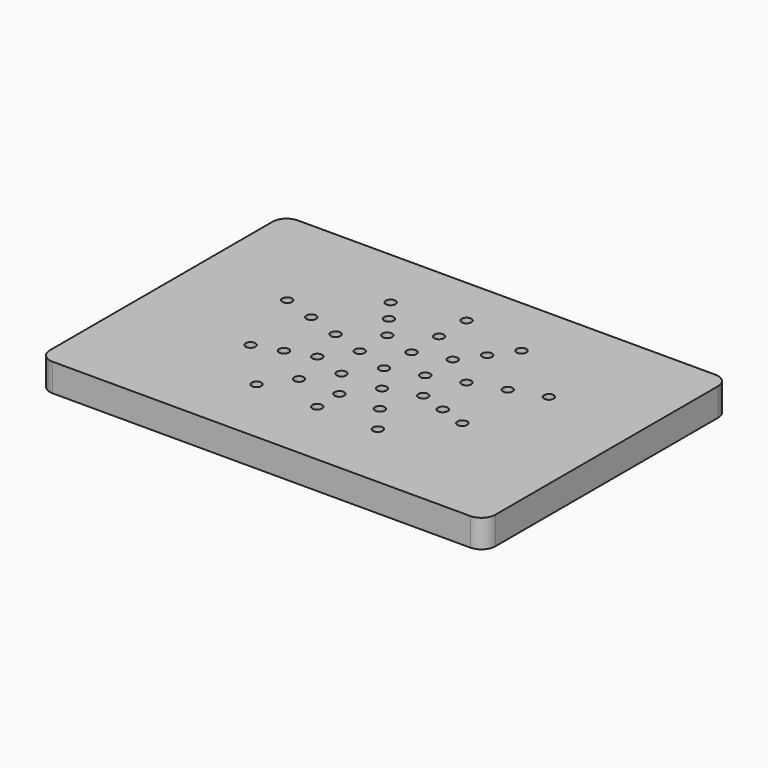
from build123d import *

# Parameters (mm, degrees)
F1_DEPTH = 6.35
F2_DEPTH = 12.7
F4_D     = 8.89
F4_DEPTH = 12.7
F4_TIP   = 2.6708254516


# Not quite as in the source:
# - a feature names something its author has since deleted; it is built from what else it names


with BuildPart() as f1:
    # F0 (on Top) → F1 (new body)
    with BuildSketch(Plane.XY):
        with BuildLine():
            Line((190.5, 139.7), (0, 139.7))
            Line((0, 139.7), (-190.5, 139.7))
            ThreePointArc((-190.5, 139.7), (-199.4802561211, 135.9802561211), (-203.2, 127))
            Line((-203.2, 127), (-203.2, 0))
            Line((-203.2, 0), (-203.2, -127))
            ThreePointArc((-203.2, -127), (-199.4802561211, -135.9802561211), (-190.5, -139.7))
            Line((-190.5, -139.7), (0, -139.7))
            Line((0, -139.7), (190.5, -139.7))
            ThreePointArc((190.5, -139.7), (199.4802561211, -135.9802561211), (203.2, -127))
            Line((203.2, -127), (203.2, 0))
            Line((203.2, 0), (203.2, 127))
            ThreePointArc((203.2, 127), (199.4802561211, 135.9802561211), (190.5, 139.7))
        make_face()
        with BuildLine():
            ThreePointArc((177.8, 127), (186.7802561211, 123.2802561211), (190.5, 114.3))
            Line((190.5, 114.3), (190.5, -114.3))
            ThreePointArc((190.5, -114.3), (186.7802561211, -123.2802561211), (177.8, -127))
            Line((177.8, -127), (-177.8, -127))
            ThreePointArc((-177.8, -127), (-186.7802561211, -123.2802561211), (-190.5, -114.3))
            Line((-190.5, -114.3), (-190.5, 114.3))
            ThreePointArc((-190.5, 114.3), (-186.7802561211, 123.2802561211), (-177.8, 127))
            Line((-177.8, 127), (177.8, 127))
        make_face(mode=Mode.SUBTRACT)
        with BuildLine():
            Line((190.5, -114.3), (190.5, 114.3))
            ThreePointArc((190.5, 114.3), (186.7802561211, 123.2802561211), (177.8, 127))
            Line((177.8, 127), (-177.8, 127))
            ThreePointArc((-177.8, 127), (-186.7802561211, 123.2802561211), (-190.5, 114.3))
            Line((-190.5, 114.3), (-190.5, -114.3))
            ThreePointArc((-190.5, -114.3), (-186.7802561211, -123.2802561211), (-177.8, -127))
            Line((-177.8, -127), (177.8, -127))
            ThreePointArc((177.8, -127), (186.7802561211, -123.2802561211), (190.5, -114.3))
        make_face()
    extrude(amount=F1_DEPTH)

    # F0 (on Top) → F2 (join)
    with BuildSketch(Plane.XY):
        with BuildLine():
            Line((190.5, 139.7), (0, 139.7))
            Line((0, 139.7), (-190.5, 139.7))
            ThreePointArc((-190.5, 139.7), (-199.4802561211, 135.9802561211), (-203.2, 127))
            Line((-203.2, 127), (-203.2, 0))
            Line((-203.2, 0), (-203.2, -127))
            ThreePointArc((-203.2, -127), (-199.4802561211, -135.9802561211), (-190.5, -139.7))
            Line((-190.5, -139.7), (0, -139.7))
            Line((0, -139.7), (190.5, -139.7))
            ThreePointArc((190.5, -139.7), (199.4802561211, -135.9802561211), (203.2, -127))
            Line((203.2, -127), (203.2, 0))
            Line((203.2, 0), (203.2, 127))
            ThreePointArc((203.2, 127), (199.4802561211, 135.9802561211), (190.5, 139.7))
        make_face()
        with BuildLine():
            ThreePointArc((177.8, 127), (186.7802561211, 123.2802561211), (190.5, 114.3))
            Line((190.5, 114.3), (190.5, -114.3))
            ThreePointArc((190.5, -114.3), (186.7802561211, -123.2802561211), (177.8, -127))
            Line((177.8, -127), (-177.8, -127))
            ThreePointArc((-177.8, -127), (-186.7802561211, -123.2802561211), (-190.5, -114.3))
            Line((-190.5, -114.3), (-190.5, 114.3))
            ThreePointArc((-190.5, 114.3), (-186.7802561211, 123.2802561211), (-177.8, 127))
            Line((-177.8, 127), (177.8, 127))
        make_face(mode=Mode.SUBTRACT)
    extrude(amount=F2_DEPTH)

    # F4
    with Locations(Plane(origin=(0, 0, 0), x_dir=(1, 0, 0), z_dir=(0, 0, -1))):
        with Locations((18.4541802113, 25.4), (-18.4541802113, 25.4), (-29.8594908165, -9.7019366858), (0, -31.3961266285), (29.8594908165, -9.7019366858), (0, 0), (-36.9083604227, 50.8), (0, 50.8), (36.9083604227, 50.8), (59.7189816329, -19.4038733715), (0, -62.792253257), (-59.7189816329, -19.4038733715), (-72.4705065417, 23.5470949714), (-55.362540634, 76.2), (0, 76.2), (55.362540634, 76.2), (72.4705065417, 23.5470949714), (89.5784724494, -29.1058100573), (44.7892362247, -61.6470949714), (0, -94.1883798855), (-44.7892362247, -61.6470949714), (-89.5784724494, -29.1058100573), (-48.3136710278, 15.6980633142), (-29.8594908165, -41.0980633142), (29.8594908165, -41.0980633142), (48.3136710278, 15.6980633142), (-96.6273420556, 31.3961266285), (-119.4379632658, -38.807746743), (-59.7189816329, -82.1961266285), (59.7189816329, -82.1961266285), (119.4379632658, -38.807746743), (96.6273420556, 31.3961266285)):
            Hole(F4_D / 2, depth=F4_DEPTH)
            with Locations((0, 0, -(F4_DEPTH + F4_TIP / 2))):  # 118° drill point
                Cone(0, F4_D / 2, F4_TIP, mode=Mode.SUBTRACT)

    # F5: F1 across face


with BuildPart() as f1_1:
    add(f1.part)
    add(f1.part.mirror(Plane.XY.offset(12.7)))


solid = f1_1.part
